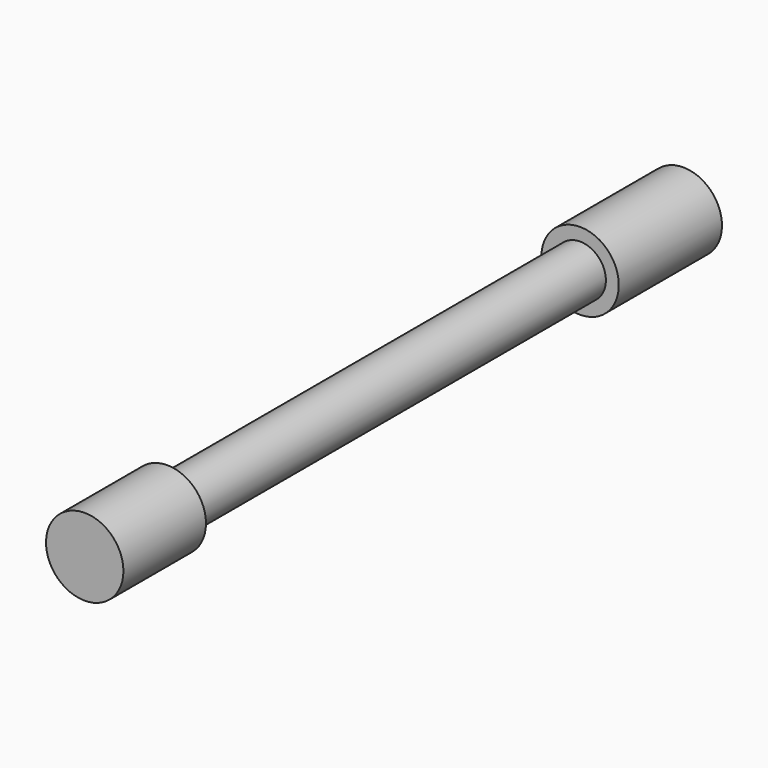
from build123d import *

# Parameters (mm, degrees)
F0_R     = 5
F1_DEPTH = 100
F2_R     = 7.5
F2_R_2   = 5
F3_DEPTH = 20
F4_R     = 7.5
F4_R_2   = 5
F5_DEPTH = 25


with BuildPart() as f1:
    # F0 (on Front) → F1 (new body)
    with BuildSketch(Plane.XZ):
        Circle(F0_R)
    extrude(amount=F1_DEPTH)

    # F2 (on face) → F3 (join)
    with BuildSketch(Plane.XZ.offset(100)):
        Circle(F2_R)
        Circle(F2_R_2, mode=Mode.SUBTRACT)
        Circle(F2_R_2)
    extrude(amount=F3_DEPTH)

    # F4 (on face) → F5 (join)
    with BuildSketch(Plane(origin=(0, 0, 0), x_dir=(-1, 0, 0), z_dir=(0, 1, 0))):
        Circle(F4_R)
        Circle(F4_R_2, mode=Mode.SUBTRACT)
        Circle(F4_R_2)
    extrude(amount=F5_DEPTH)


solid = f1.part
